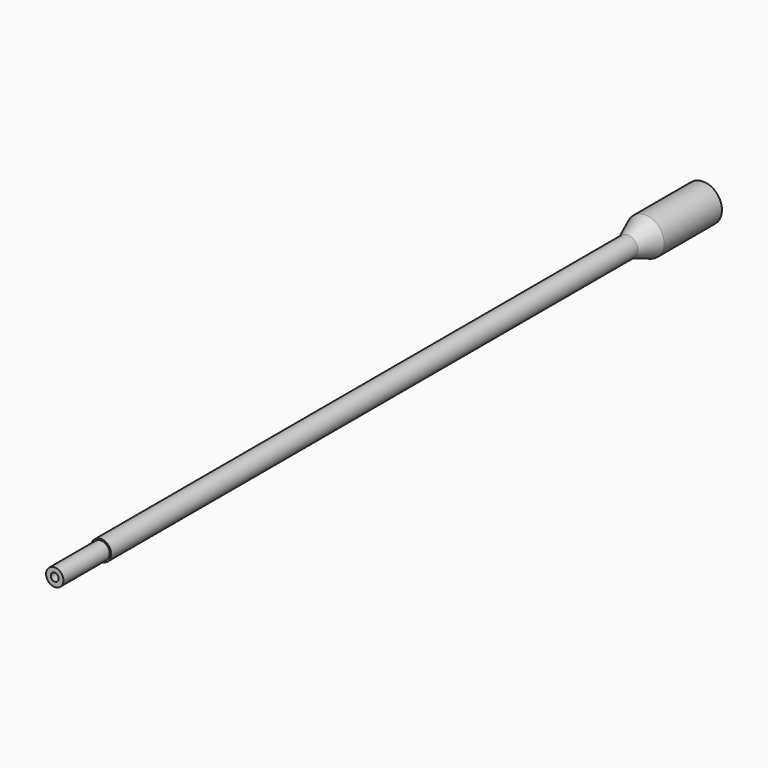
from build123d import *

# Parameters (mm, degrees)
F0_R         = 7
F1_DEPTH     = 560
F2_R         = 7
F2_R_2       = 6
F3_DEPTH     = 40
F4_R         = 2.75
F5_DEPTH     = 560.001
F6_R         = 1.75
F7_DEPTH     = 10
F8_R         = 13
F8_R_2       = 7
F9_DEPTH     = 70
F10_S5_R     = 7
F10_T6_DEPTH = 22


# Not quite as in the source:
# - a fillet or chamfer that OpenCascade refuses, or shapes differently, is made with other operations: its cross-section is extruded or revolved along the edge and cut away or added


with BuildPart() as f1:
    # F0 (on Front) → F1 (new body)
    with BuildSketch(Plane.XZ):
        Circle(F0_R)
    extrude(amount=-F1_DEPTH)

    # F2 (on face) → F3 (cut)
    with BuildSketch(Plane.XZ):
        Circle(F2_R)
        Circle(F2_R_2, mode=Mode.SUBTRACT)
    extrude(amount=-F3_DEPTH, mode=Mode.SUBTRACT)

    # F4 (on face) → F5 (cut, through all)
    with BuildSketch(Plane.XZ):
        Circle(F4_R)
    extrude(amount=-F5_DEPTH, mode=Mode.SUBTRACT)

    # F6 (on Top) → F7 (cut)
    with BuildSketch(Plane.XY):
        with Locations((0, 8)):
            Circle(F6_R)
    extrude(amount=-F7_DEPTH, mode=Mode.SUBTRACT)

    # F8 (on face) → F9 (join)
    with BuildSketch(Plane(origin=(0, 560, 0), x_dir=(-1, 0, 0), z_dir=(0, 1, 0))):
        Circle(F8_R)
        Circle(F8_R_2, mode=Mode.SUBTRACT)
    extrude(amount=-F9_DEPTH)

    # F10: chamfer of 20 x 8 on 1 edges, made by hand


with BuildPart() as f10_tool2:
    # F10_s3 → F10_t4 (revolve)
    with BuildSketch(Plane.XY):
        Polygon((-5, 490), (-13, 510), (-13, 490), align=None)
    revolve(axis=Axis((0, 490, 0), (0, 1, 0)))

    # F10_s5 → F10_t6 (cut, symmetric)
    with BuildSketch(Plane.XZ.offset(-500)):
        Circle(F10_S5_R)
    extrude(amount=F10_T6_DEPTH, both=True, mode=Mode.SUBTRACT)


with BuildPart() as f1_1:
    add(f1.part)

    # F10_t1: cut F10_tool2
    add(f10_tool2.part, mode=Mode.SUBTRACT)


solid = f1_1.part
